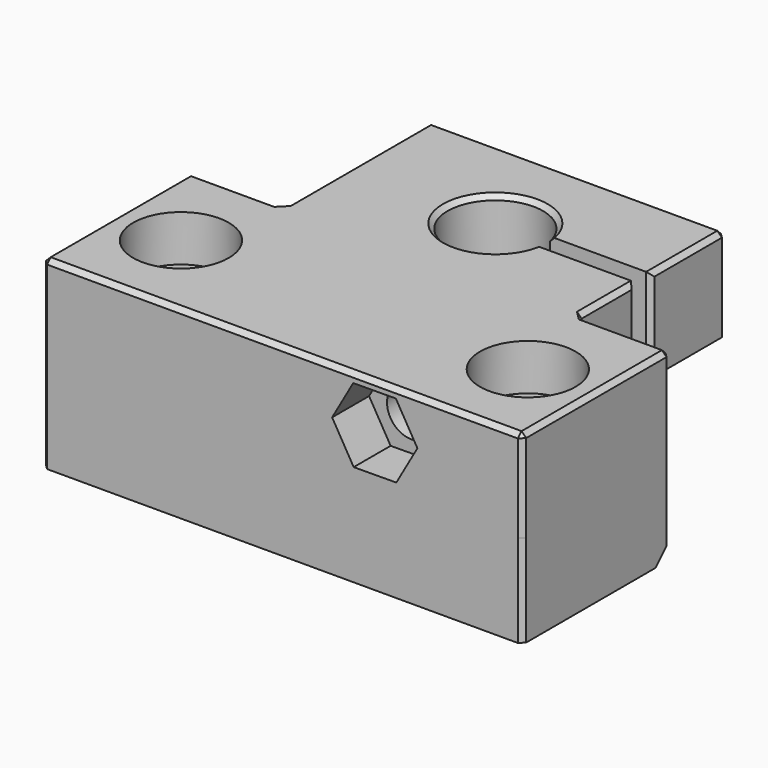
from build123d import *

# Parameters (mm, degrees)
F0_R      = 5.175
F1_DEPTH  = 10
F0_R_2    = 2.675
F2_DEPTH  = 5
F3_DEPTH  = 5
F4_R      = 2.675
F5_DEPTH  = 40
F6_DEPTH  = 5
F7_R      = 4
F7_R_2    = 2.675
F8_DEPTH  = 5
F9_SIZE   = 0.5
F10_DEPTH = 10
F11_DEPTH = 10
F12_SIZE  = 0.49999
F13_SIZE  = 2


# Not quite as in the source:
# - a fillet or chamfer is up to 0.001 mm smaller than in the source, because OpenCascade refuses the exact size


with BuildPart() as f1:
    # F0 (on Top) → F1 (new body)
    with BuildSketch(Plane.XY):
        with BuildLine():
            Line((14.923914507, 11.175), (-17.076085493, 11.175))
            Line((-17.076085493, 11.175), (-17.076085493, -8.825))
            Line((-17.076085493, -8.825), (14.923914507, -8.825))
            Line((14.923914507, -8.825), (14.923914507, -1.035))
            Line((14.923914507, -1.035), (3.9943582746, -1.035))
            ThreePointArc((3.9943582746, -1.035), (-6.251085493, 0), (3.9943582746, 1.035))
            Line((3.9943582746, 1.035), (14.923914507, 1.035))
            Line((14.923914507, 1.035), (14.923914507, 11.175))
        make_face()
        Polygon((14.923914507, -8.825), (-17.076085493, -8.825), (-27.076085493, -8.825), (-27.076085493, -28.825), (-17.076085493, -28.825), (14.923914507, -28.825), (24.923914507, -28.825), (24.923914507, -8.825), align=None)
        with Locations((-19.901085493, -19.0323841524)):
            Circle(F0_R, mode=Mode.SUBTRACT)
        with Locations((17.748914507, -19.1356375643)):
            Circle(F0_R, mode=Mode.SUBTRACT)
    extrude(amount=F1_DEPTH)

    # F0 (on Top) → F2 (join)
    with BuildSketch(Plane.XY):
        with Locations((-19.901085493, -19.0323841524)):
            Circle(F0_R)
        with Locations((-19.901085493, -19.0323841524)):
            Circle(F0_R_2, mode=Mode.SUBTRACT)
    extrude(amount=F2_DEPTH)

    # F0 (on Top) → F3 (join)
    with BuildSketch(Plane.XY):
        with Locations((17.748914507, -19.1356375643)):
            Circle(F0_R)
        with Locations((17.748914507, -19.1356375643)):
            Circle(F0_R_2, mode=Mode.SUBTRACT)
    extrude(amount=F3_DEPTH)

    # F4 (on face) → F5 (cut)
    with BuildSketch(Plane.XZ.offset(28.825)):
        with Locations((8.923914507, 5)):
            Circle(F4_R)
    extrude(amount=-F5_DEPTH, mode=Mode.SUBTRACT)

    # F4 (on face) → F6 (cut)
    with BuildSketch(Plane.XZ.offset(28.825)):
        Polygon((4.3052091527, 4.9700971099), (6.6404584923, 0.9851323855), (11.2591638467, 1.0150352756), (13.5426198614, 5.0299028901), (11.2073705218, 9.0148676145), (6.5886651674, 8.9849647244), align=None)
        with Locations((8.923914507, 5)):
            Circle(F4_R, mode=Mode.SUBTRACT)
    extrude(amount=-F6_DEPTH, mode=Mode.SUBTRACT)

    # F7 (on face) → F8 (cut)
    with BuildSketch(Plane(origin=(0, 11.175, 0), x_dir=(-1, 0, 0), z_dir=(0, 1, 0))):
        with Locations((-8.923914507, 5)):
            Circle(F7_R)
        with Locations((-8.923914507, 5)):
            Circle(F7_R_2, mode=Mode.SUBTRACT)
    extrude(amount=-F8_DEPTH, mode=Mode.SUBTRACT)

    # F9
    f9_edges = [f1.edges().sort_by_distance(p)[0] for p in [
        (-27.076085, -18.825, 10),
        (-22.076085, -8.825, 10),
        (-17.076085, 1.175, 10),
        (-1.076085, 11.175, 10),
        (14.923915, 6.105, 10),
        (14.923915, -4.93, 10),
        (19.923915, -8.825, 10),
        (24.923915, -18.825, 10),
        (24.923915, -8.825, 5),
        (14.923915, -8.825, 5),
        (14.923915, -1.035, 5),
        (14.923915, 1.035, 5),
        (14.923915, 11.175, 5),
        (-17.076085, 11.175, 5),
        (-17.076085, -8.825, 5),
        (-27.076085, -8.825, 5),
        (-27.076085, -28.825, 5),
        (24.923915, -28.825, 5),
        (-6.251085, 0, 10),
        (-1.076085, -28.825, 10),
        (-6.251085, 0, 0),
        (-1.076085, 11.175, 0),
    ]]
    chamfer(f9_edges, length=F9_SIZE)

    # F0 (on Top) → F10 (join)
    with BuildSketch(Plane.XY):
        Polygon((14.923914507, -8.825), (-17.076085493, -8.825), (-27.076085493, -8.825), (-27.076085493, -28.825), (-17.076085493, -28.825), (14.923914507, -28.825), (24.923914507, -28.825), (24.923914507, -8.825), align=None)
        with Locations((-19.901085493, -19.0323841524)):
            Circle(F0_R, mode=Mode.SUBTRACT)
        with Locations((17.748914507, -19.1356375643)):
            Circle(F0_R, mode=Mode.SUBTRACT)
    extrude(amount=-F10_DEPTH)

    # F0 (on Top) → F11 (join)
    with BuildSketch(Plane.XY):
        with Locations((17.748914507, -19.1356375643)):
            Circle(F0_R)
        with Locations((17.748914507, -19.1356375643)):
            Circle(F0_R_2, mode=Mode.SUBTRACT)
        with Locations((-19.901085493, -19.0323841524)):
            Circle(F0_R)
        with Locations((-19.901085493, -19.0323841524)):
            Circle(F0_R_2, mode=Mode.SUBTRACT)
    extrude(amount=-F11_DEPTH)

    # F12 (size 0.5 in the source; OpenCascade refuses exactly that, so slightly less here)
    f12_edges = [f1.edges().sort_by_distance(p)[0] for p in [
        (24.923915, -8.825, -5),
        (-27.076085, -8.825, -5),
        (24.923915, -28.825, -5),
        (-27.076085, -28.825, -5),
    ]]
    chamfer(f12_edges, length=F12_SIZE)

    # F13
    f13_edges = [f1.edges().sort_by_distance(p)[0] for p in [
        (-1.076085, -8.825, -10),
    ]]
    chamfer(f13_edges, length=F13_SIZE)


solid = f1.part
